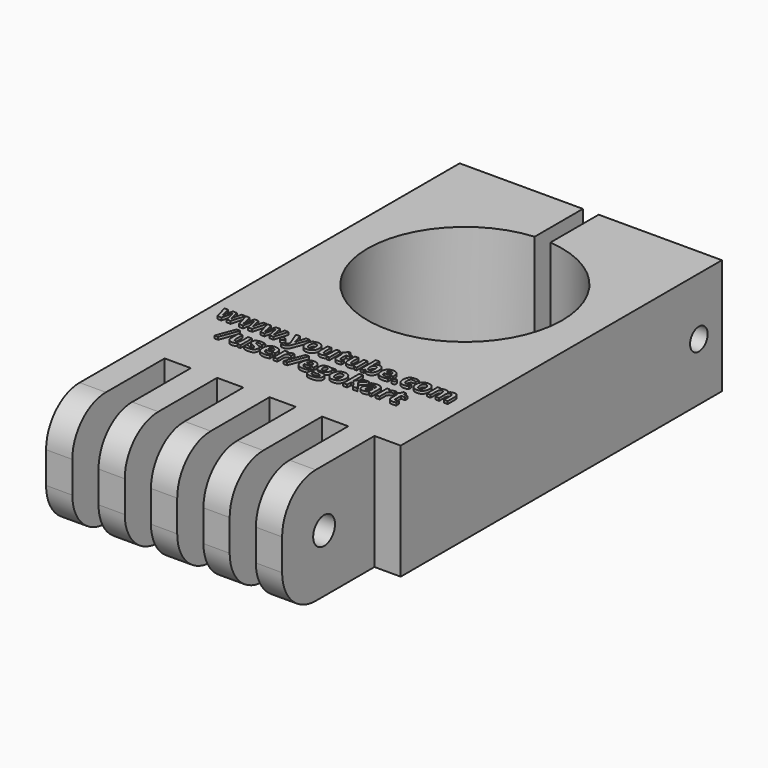
from build123d import *

# Parameters (mm, degrees)
F0_W           = 50
F0_H           = 98.55
F0_R           = 18.55
F1_DEPTH       = 22
F3_R           = 8
F2_W           = 5
F2_H           = 22
F4_DEPTH       = 22
F5_W           = 3
F5_H           = 22
F6_DEPTH       = 18
F7_R           = 2.1
F7_R_2         = 2.6
F8_DEPTH       = 50.001
F9_TEXT_SIZE   = 4.7853250033
F9_TEXT_SIZE_2 = 5.0393700787
F10_DEPTH      = 0.5


# Not quite as in the source:
# - Text() gives the source's letters only with a copy of the font that has no kerning and outlines rounded to 1/6400 em; it was checked with that copy


with BuildPart() as f1:
    # F0 (on Top) → F1 (new body)
    with BuildSketch(Plane.XY):
        with Locations((0, -19.275)):
            Rectangle(F0_W, F0_H)
        Circle(F0_R, mode=Mode.SUBTRACT)
    extrude(amount=F1_DEPTH)

    # F3
    f3_edges = [f1.edges().sort_by_distance(p)[0] for p in [
        (0, -68.55, 22),
        (0, -68.55, 0),
    ]]
    fillet(f3_edges, radius=F3_R)

    # F2 (on face) → F4 (cut)
    with BuildSketch(Plane.XZ.offset(68.55)):
        with Locations((-17.5, 11)):
            Rectangle(F2_W, F2_H)
        with Locations((-7.5, 11)):
            Rectangle(F2_W, F2_H)
        with Locations((2.5, 11)):
            Rectangle(F2_W, F2_H)
        with Locations((12.5, 11)):
            Rectangle(F2_W, F2_H)
        with Locations((22.5, 11)):
            Rectangle(F2_W, F2_H)
    extrude(amount=-F4_DEPTH, mode=Mode.SUBTRACT)

    # F5 (on face) → F6 (cut)
    with BuildSketch(Plane(origin=(0, 30, 0), x_dir=(-1, 0, 0), z_dir=(0, 1, 0))):
        with Locations((0, 11)):
            Rectangle(F5_W, F5_H)
    extrude(amount=-F6_DEPTH, mode=Mode.SUBTRACT)

    # F7 (on face) → F8 (cut, through all)
    with BuildSketch(Plane.YZ.offset(25)):
        with Locations((24.5, 11)):
            Circle(F7_R)
        with Locations((-58.55, 11)):
            Circle(F7_R_2)
    extrude(amount=-F8_DEPTH, mode=Mode.SUBTRACT)

    # F9 (on face) → F10 (join)
    with BuildSketch(Plane.XY.offset(22)):
        with Locations((-22.5839550938, -31.7284227517)):
            Text('www.youtube.com', F9_TEXT_SIZE, font='Open Sans', font_style=FontStyle.BOLD, text_align=(TextAlign.LEFT, TextAlign.BOTTOM))
        with Locations((-18.2500195711, -36.9078821209)):
            Text('/user/egokart', F9_TEXT_SIZE_2, font='Open Sans', font_style=FontStyle.BOLD, text_align=(TextAlign.LEFT, TextAlign.BOTTOM))
    extrude(amount=F10_DEPTH)


solid = f1.part
